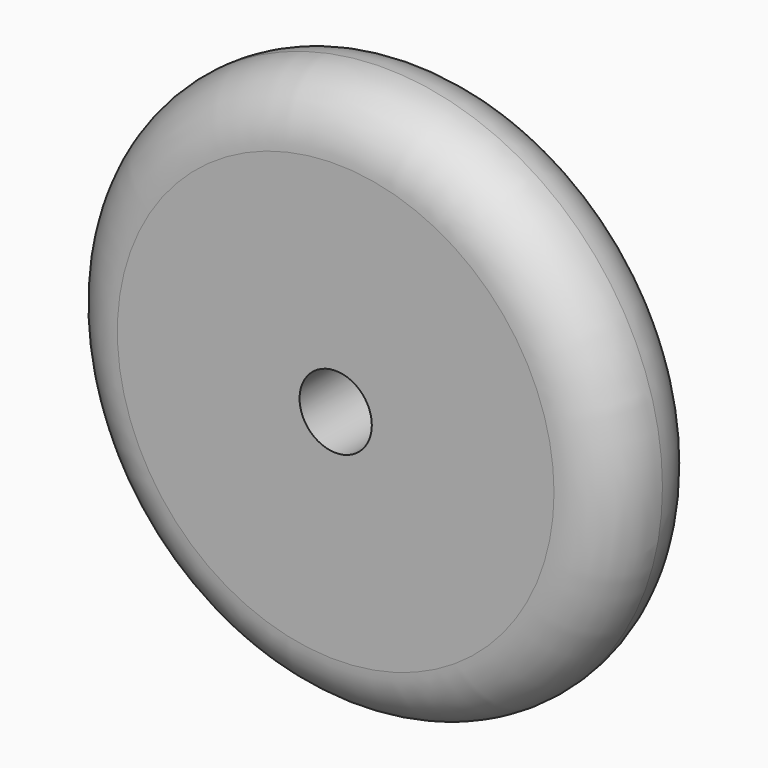
from build123d import *

# Parameters (mm, degrees)
F0_R     = 23.125
F0_R_2   = 3
F1_DEPTH = 10
F2_R     = 4.99999
F3_R     = 2


# Not quite as in the source:
# - a fillet or chamfer is up to 0.001 mm smaller than in the source, because OpenCascade refuses the exact size


with BuildPart() as f1:
    # F0 (on Front) → F1 (new body)
    with BuildSketch(Plane.XZ):
        Circle(F0_R)
        Circle(F0_R_2, mode=Mode.SUBTRACT)
    extrude(amount=F1_DEPTH)

    # F2 (radius 5 in the source; OpenCascade refuses exactly that, so slightly less here)
    f2_edges = [f1.edges().sort_by_distance(p)[0] for p in [
        (-23.125, 0, 0),
        (-23.125, -10, 0),
    ]]
    fillet(f2_edges, radius=F2_R)

    # F3
    f3_edges = [f1.edges().sort_by_distance(p)[0] for p in [
        (-3, 0, 0),
        (-18.12501, 0, 0),
    ]]
    fillet(f3_edges, radius=F3_R)


solid = f1.part
